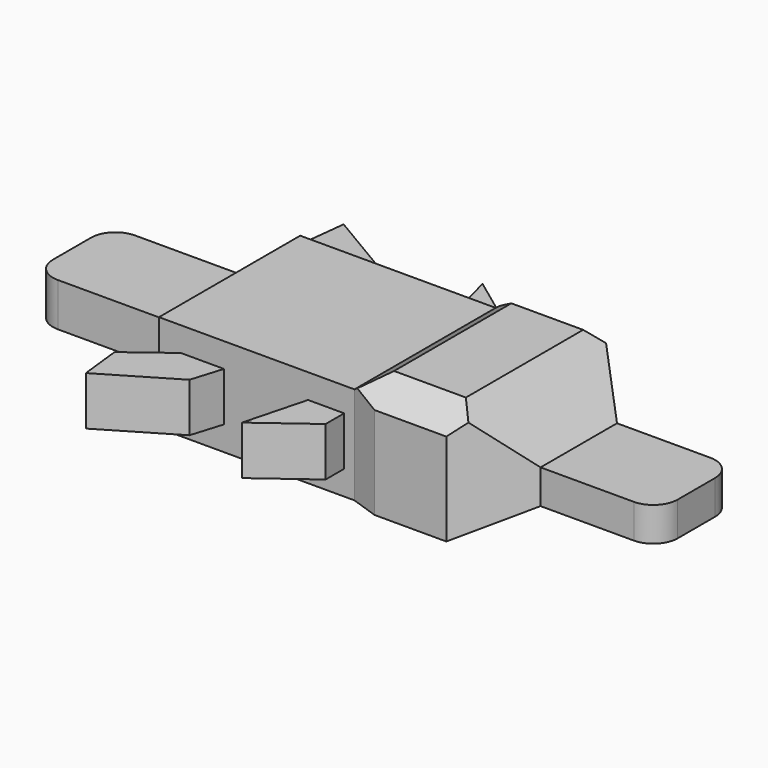
from build123d import *

# Parameters (mm, degrees)
F1_DEPTH = 20
F3_DEPTH = 43.4
F5_DEPTH = 5
F6_R     = 5
F8_SIZE  = 5


# Not quite as in the source:
# - a feature names something its author has since deleted; it is built from what else it names


with BuildPart() as f1:
    # F0 (on Front) → F1 (new body, symmetric)
    with BuildSketch(Plane.XZ):
        Polygon((20, 10), (-20, 10), (-26.2878760695, 4.5041712001), (-52.2599183023, 4.5041712001), (-52.2599183023, -4.38100053), (-26.2878760695, -4.38100053), (-20, -10), (20, -10), (40.3509177268, -10), (51.457375288, -4.1727770417), (75.5315572023, -4.1727770417), (75.5315572023, 2.809499735), (51.457375288, 2.809499735), (40.3509177268, 13.9019489288), (25.6562046707, 13.9019489288), align=None)
    extrude(amount=F1_DEPTH, both=True)

    # F2 (on face) → F3 (cut, symmetric)
    with BuildSketch(Plane.XY.offset(10)):
        Polygon((-20, 18.0594865233), (20, 18.0594865233), (25.6562046707, 20), (40.3509177268, 20), (51.457375288, 9.7775636241), (82.4265927076, 9.7775636241), (82.4265927076, -9.7775636241), (51.457375288, -9.7775636241), (40.3509177268, -20), (25.6562046707, -20), (20, -18.0594865233), (-20, -18.0594865233), (-26.2878760695, -9.8739182577), (-73.8637112081, -9.8739182577), (-73.8637112081, -40.0371998549), (108.4082424641, -42.2960631549), (105.6976020336, 36.3123118877), (-67.5570517778, 60.9338954091), (-73.8637112081, 9.8739182577), (-26.2878760695, 9.8739182577), align=None)
    extrude(amount=F3_DEPTH, both=True, mode=Mode.SUBTRACT)

    # F4 (on Top) → F5 (join, symmetric)
    with BuildSketch(Plane.XY):
        Polygon((17.8880691528, -22.8056833148), (17.8880691528, -14.7547144443), (11.4664630964, -14.3713355064), (7.1534435265, -30.7608079165), align=None)
        Polygon((-5.6897685863, -14.7547144443), (-11.1529268324, -14.7547144443), (-23.9961370826, -24.4350470603), (-23.0376925319, -32.9652391374), (-8.6609609425, -24.4350470603), align=None)
        Polygon((-8.6609609425, 24.4350470603), (-23.0376925319, 32.9652391374), (-23.9961370826, 24.4350470603), (-11.1529268324, 14.7547144443), (-5.6897685863, 14.7547144443), align=None)
        Polygon((7.1534435265, 30.7608079165), (11.4664630964, 14.3713355064), (17.8880691528, 14.7547144443), (17.8880691528, 22.8056833148), align=None)
    extrude(amount=F5_DEPTH, both=True)

    # F6
    f6_edges = [f1.edges().sort_by_distance(p)[0] for p in [
        (-52.259918, 9.873918, 0.061585),
        (75.531557, 9.777564, -0.681639),
        (75.531557, -9.777564, -0.681639),
        (-52.259918, -9.873918, 0.061585),
    ]]
    fillet(f6_edges, radius=F6_R)

    # F8
    f8_edges = [f1.edges().sort_by_distance(p)[0] for p in [
        (33.003561, -20, 13.901949),
        (33.003561, 20, 13.901949),
    ]]
    chamfer(f8_edges, length=F8_SIZE)


solid = f1.part
